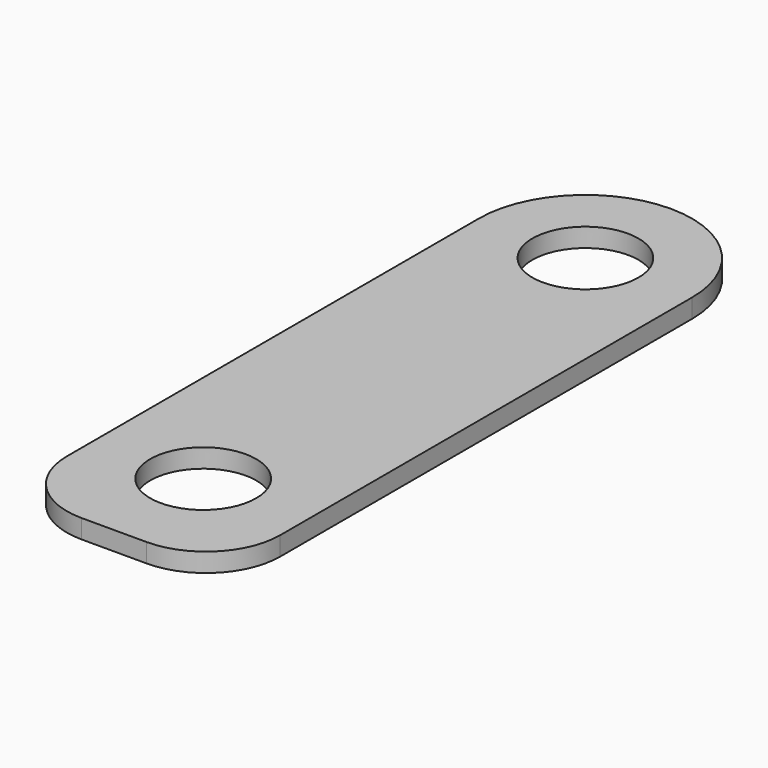
from build123d import *

# Parameters (mm, degrees)
F0_R     = 14.2875
F1_DEPTH = 5.08


# Not quite as in the source:
# - a feature names something its author has since deleted; it is built from what else it names


with BuildPart() as f1:
    # F0 (on Top) → F1 (new body)
    with BuildSketch(Plane.XY):
        with BuildLine():
            ThreePointArc((0, 20), (5.8578643763, 5.8578643763), (20, 0))
            Line((20, 0), (37.5, 0))
            ThreePointArc((37.5, 0), (51.6421356237, 5.8578643763), (57.5, 20))
            Line((57.5, 20), (57.5, 158.715))
            ThreePointArc((57.5, 158.715), (28.75, 187.465), (0, 158.715))
            Line((0, 158.715), (0, 20))
        make_face()
        with Locations((28.75, 30)):
            Circle(F0_R, mode=Mode.SUBTRACT)
        with Locations((28.75, 158.715)):
            Circle(F0_R, mode=Mode.SUBTRACT)
    extrude(amount=F1_DEPTH)


solid = f1.part
